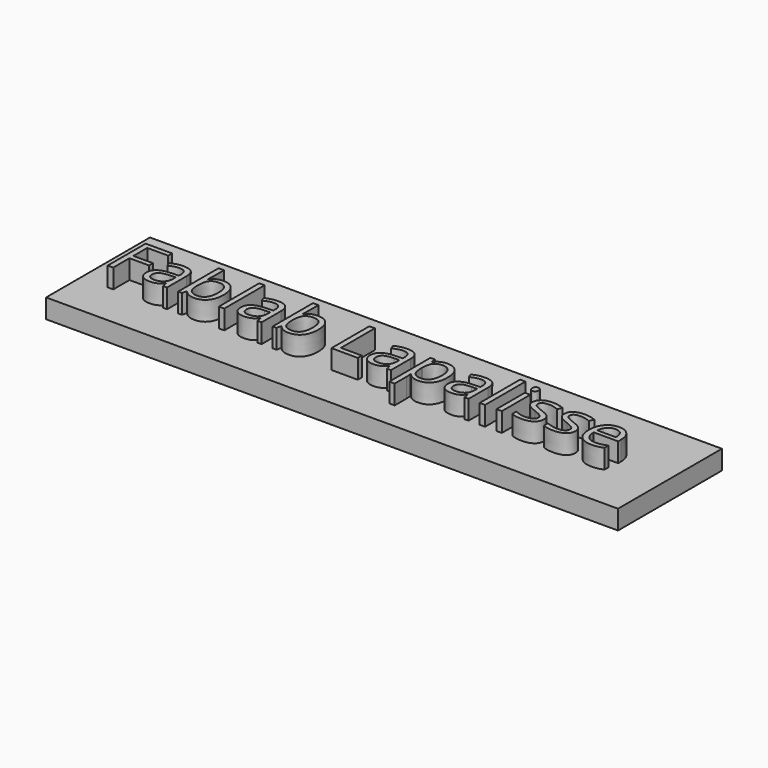
from build123d import *

# Parameters (mm, degrees)
F0_TEXT_SIZE = 87.700297849
F1_DEPTH     = 25.4
F2_W         = 755.02050668
F2_H         = 171.4823693037
F3_DEPTH     = 25.4


# Not quite as in the source:
# - Text() gives the source's letters only with a copy of the font that has no kerning and outlines rounded to 1/6400 em; it was checked with that copy


with BuildPart() as f1:
    # F0 (on Top) → F1 (new body)
    with BuildSketch(Plane.XY):
        with Locations((-64.6611452103, -30.5031277239)):
            Text('Fablab Lapalisse', F0_TEXT_SIZE, font='Open Sans', text_align=(TextAlign.LEFT, TextAlign.BOTTOM))
    extrude(amount=F1_DEPTH)


with BuildPart() as f3:
    # F2 (on Top) → F3 (new body)
    with BuildSketch(Plane.XY):
        with Locations((285.8281098306, -1.9932463765)):
            Rectangle(F2_W, F2_H)
    extrude(amount=-F3_DEPTH)


solid = Compound([f1.part, f3.part])
